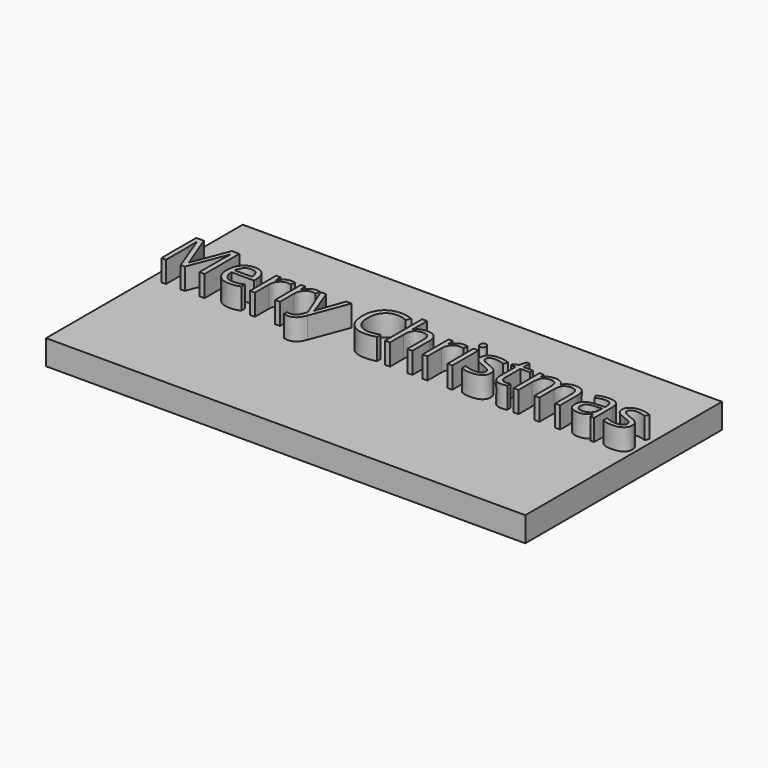
from build123d import *

# Parameters (mm, degrees)
F0_W         = 245.2980130911
F0_H         = 125.8012056351
F1_DEPTH     = 12.7
F2_W         = 233.8354885578
F2_H         = 113.76555264
F3_DEPTH     = 11.684
F5_DEPTH     = 12.7
F6_R         = 10.4661084843
F6_W         = 8.1836208701
F6_H         = 17.311509233
F6_R_2       = 9.3100126353
F7_DEPTH     = 1.524
F8_DEPTH     = 1.27
F9_TEXT_SIZE = 31.2525199474
F10_DEPTH    = 10.922


# Not quite as in the source:
# - Text() gives the source's letters only with a copy of the font that has no kerning and outlines rounded to 1/6400 em; it was checked with that copy


with BuildPart() as f1:
    # F0 (on Top) → F1 (new body)
    with BuildSketch(Plane.XY):
        Rectangle(F0_W, F0_H)
    extrude(amount=F1_DEPTH)

    # F2 (on Top) → F3 (cut)
    with BuildSketch(Plane.XY):
        Rectangle(F2_W, F2_H)
    extrude(amount=F3_DEPTH, mode=Mode.SUBTRACT)

    # F4 (on Top) → F5 (join)
    with BuildSketch(Plane.XY):
        with BuildLine():
            ThreePointArc((48.3923600833, -16.7432173529), (82.3977539228, -29.0182551065), (103.9612469749, 0))
            ThreePointArc((103.9612469749, 0), (83.2103534484, 28.7608954329), (49.3736577324, 18.1370208442))
            ThreePointArc((49.3736577324, 18.1370208442), (43.3595213626, 0.8522959064), (48.3923600833, -16.7432173529))
        make_face()
        with BuildLine():
            ThreePointArc((48.3923600833, -16.7432173529), (43.3595213626, 0.8522959064), (49.3736577324, 18.1370208442))
            Line((49.3736577324, 18.1370208442), (47.5051735648, 24.4088333072))
            ThreePointArc((47.5051735648, 24.4088333072), (46.3842237042, 26.5548459463), (44.5415252482, 28.1253112396))
            Line((44.5415252482, 28.1253112396), (5.1208234912, 50.3827026103))
            ThreePointArc((5.1208234912, 50.3827026103), (-4.7359791399, 46.1018792877), (0.6272320354, 36.7896307774))
            Line((0.6272320354, 36.7896307774), (7.7651561313, 32.2095985294))
            ThreePointArc((7.7651561313, 32.2095985294), (10.2595924764, 24.5776868842), (3.283162905, 20.6030525016))
            Line((3.283162905, 20.6030525016), (-40.5268037766, 27.9681689954))
            Line((-40.5268037766, 27.9681689954), (-40.3414088484, 40.5109878393))
            ThreePointArc((-40.3414088484, 40.5109878393), (-42.1675283551, 45.061660664), (-46.6907152981, 46.9548366964))
            Line((-46.6907152981, 46.9548366964), (-57.4775928795, 46.9548366964))
            ThreePointArc((-57.4775928795, 46.9548366964), (-61.9677209401, 45.0949647569), (-63.8275928795, 40.6048366964))
            Line((-63.8275928795, 40.6048366964), (-63.8275928795, 22.7411282346))
            ThreePointArc((-63.8275928795, 22.7411282346), (-62.82720457, 19.3199946854), (-60.1412449232, 16.9768019261))
            Line((-60.1412449232, 16.9768019261), (-35.8922111882, 5.7715049308))
            ThreePointArc((-35.8922111882, 5.7715049308), (-32.2058639443, 0.0041704732), (-35.8976737858, -5.7596687719))
            Line((-35.8976737858, -5.7596687719), (-61.2502071589, -17.4457481903))
            ThreePointArc((-61.2502071589, -17.4457481903), (-63.940008129, -19.7889281783), (-64.9420177129, -23.2125955845))
            Line((-64.9420177129, -23.2125955845), (-64.9420177129, -44.2485610924))
            ThreePointArc((-64.9420177129, -44.2485610924), (-63.0821457734, -48.7386891529), (-58.5920177129, -50.5985610924))
            Line((-58.5920177129, -50.5985610924), (-47.7323308587, -50.5985610924))
            ThreePointArc((-47.7323308587, -50.5985610924), (-43.2422027982, -48.7386891529), (-41.3823308587, -44.2485610924))
            Line((-41.3823308587, -44.2485610924), (-41.3823308587, -24.1459061422))
            Line((-41.3823308587, -24.1459061422), (4.1756192101, -21.8905627128))
            ThreePointArc((4.1756192101, -21.8905627128), (10.626318102, -26.6009009091), (7.3674048887, -33.8932453048))
            Line((7.3674048887, -33.8932453048), (0, -37.638887763))
            ThreePointArc((0, -37.638887763), (-3.3965350429, -48.8966470186), (7.8394276465, -52.3646055242))
            Line((7.8394276465, -52.3646055242), (44.8107375318, -28.6225001536))
            ThreePointArc((44.8107375318, -28.6225001536), (46.7988208158, -26.5889656334), (47.6999169192, -23.891603292))
            Line((47.6999169192, -23.891603292), (48.3923600833, -16.7432173529))
        make_face()
    extrude(amount=F5_DEPTH)

    # F6 (on Top) → F7 (join)
    with BuildSketch(Plane.XY):
        with Locations((86.5033194423, -11.076820083)):
            Circle(F6_R)
        with Locations((87.1328264475, 10.9560107812)):
            Circle(F6_R)
        with BuildLine():
            Line((65.4147490859, -12.9653457552), (65.7295063138, 13.4740453213))
            ThreePointArc((65.7295063138, 13.4740453213), (58.3508849118, 0.3403176616), (65.4147490859, -12.9653457552))
        make_face()
        Polygon((45.4383455217, -14.8681579158), (41.8081507087, -8.873534156), (33.6245298386, -8.873534156), (30.0153680146, -14.8681579158), align=None)
        with Locations((37.7163402736, -0.2177795395)):
            Rectangle(F6_W, F6_H)
        Polygon((33.6245298386, 8.437975077), (41.8081507087, 8.437975077), (45.4383455217, 15.3482910246), (30.0153680146, 15.0682402349), align=None)
        with Locations((20.7195859402, 0)):
            Circle(F6_R_2)
        with Locations((-5.405053962, 0)):
            Circle(F6_R_2)
    extrude(amount=-F7_DEPTH)

    # F6 (on Top) → F8 (join)
    with BuildSketch(Plane.XY):
        with Locations((86.5033194423, -11.076820083)):
            Circle(F6_R)
        with Locations((87.1328264475, 10.9560107812)):
            Circle(F6_R)
        with BuildLine():
            Line((65.4147490859, -12.9653457552), (65.7295063138, 13.4740453213))
            ThreePointArc((65.7295063138, 13.4740453213), (58.3508849118, 0.3403176616), (65.4147490859, -12.9653457552))
        make_face()
        Polygon((45.4383455217, -14.8681579158), (41.8081507087, -8.873534156), (33.6245298386, -8.873534156), (30.0153680146, -14.8681579158), align=None)
        with Locations((37.7163402736, -0.2177795395)):
            Rectangle(F6_W, F6_H)
        Polygon((33.6245298386, 8.437975077), (41.8081507087, 8.437975077), (45.4383455217, 15.3482910246), (30.0153680146, 15.0682402349), align=None)
        with Locations((20.7195859402, 0)):
            Circle(F6_R_2)
        with Locations((-5.405053962, 0)):
            Circle(F6_R_2)
    extrude(amount=-F8_DEPTH)

    # F9 (on face) → F10 (join)
    with BuildSketch(Plane.XY.offset(12.7)):
        with Locations((-119.9437963401, 3.6667204473)):
            Text('Merry Christmas', F9_TEXT_SIZE, font='Open Sans', text_align=(TextAlign.LEFT, TextAlign.BOTTOM))
    extrude(amount=F10_DEPTH)


solid = f1.part
